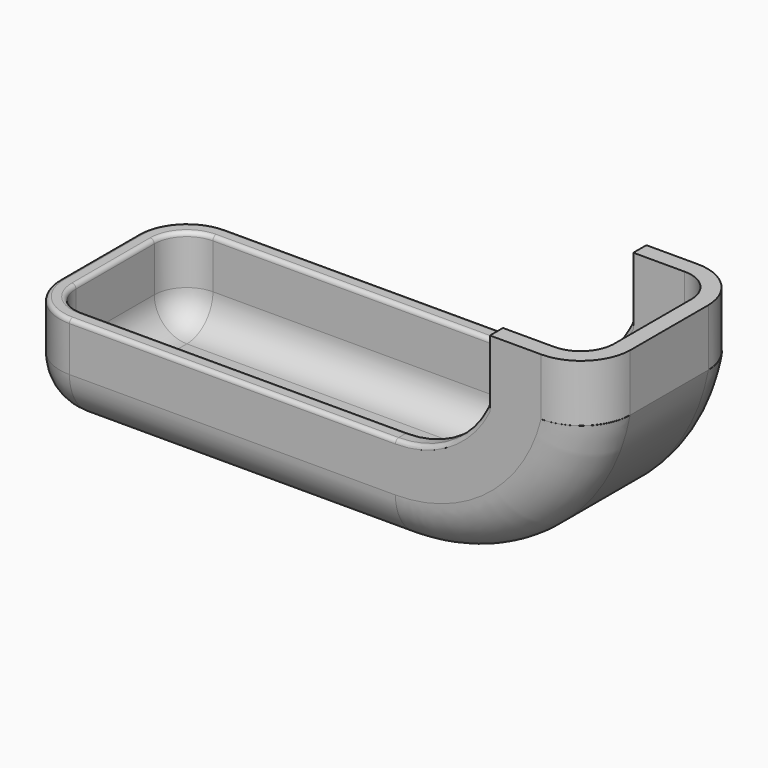
from build123d import *

# Parameters (mm, degrees)
F3_R      = 6
F4_T      = -2
F6_W      = 43.5708351433
F6_H      = 71.2567269802
F7_DEPTH  = 25.2
F9_DEPTH  = 7
F10_W     = 21.0461514253
F10_H     = 5.3538460713
F11_DEPTH = 73.3
F12_R     = 0.5


with BuildPart() as f2:
    # F2: sweep along a path in F0
    with BuildLine(Plane.XZ) as f2_path:
        Line((0, -24.4), (46, -24.4))
        ThreePointArc((46, -24.4), (61.6204993518, -18.7445992222), (70, -4.4))
    # F1 (on Right) → F2 (sweep)
    with BuildSketch(Plane.YZ):
        with BuildLine():
            Line((-6, -24.4), (6, -24.4))
            ThreePointArc((6, -24.4), (10.2426406871, -22.6426406871), (12, -18.4))
            Line((12, -18.4), (12, -12.4))
            Line((12, -12.4), (-12, -12.4))
            Line((-12, -12.4), (-12, -18.4))
            ThreePointArc((-12, -18.4), (-10.2426406871, -22.6426406871), (-6, -24.4))
        make_face()
    sweep(path=f2_path.line)

    # F3
    f3_edges = [f2.edges().sort_by_distance(p)[0] for p in [
        (0, -12, -15.4),
        (0, 10.242641, -22.642641),
        (0, 12, -15.4),
        (0, -10.242641, -22.642641),
    ]]
    fillet(f3_edges, radius=F3_R)

    # F4
    f4_openings = [f2.faces().sort_by_distance(p)[0] for p in [
        (23.307448, 0, -12.4),
        (53.938287, 0, -9.525944),
        (63.838518, 0, -3.270395),
    ]]
    offset(amount=F4_T, openings=f4_openings)

    # F6 (on face) → F7 (cut)
    with BuildSketch(Plane.XY.offset(-4.4)):
        with Locations((56.7423906177, -0.4439689219)):
            Rectangle(F6_W, F6_H)
    extrude(amount=F7_DEPTH, mode=Mode.SUBTRACT)

    # F8 (on face) → F9 (join)
    with BuildSketch(Plane.XY.offset(-4.4)):
        with BuildLine():
            Line((63.8661691473, 12), (57.593101397, 12))
            Line((57.593101397, 12), (57.593101397, 10))
            Line((57.593101397, 10), (63.8661691473, 10))
            ThreePointArc((63.8661691473, 10), (66.7292527517, 8.8342023924), (67.9636062613, 6))
            Line((67.9636062613, 6), (67.9636062613, -6))
            ThreePointArc((67.9636062613, -6), (66.7292527517, -8.8342023924), (63.8661691473, -10))
            Line((63.8661691473, -10), (57.593101397, -10))
            Line((57.593101397, -10), (57.593101397, -12))
            Line((57.593101397, -12), (63.8661691473, -12))
            ThreePointArc((63.8661691473, -12), (68.1563871176, -10.250588481), (70, -6))
            Line((70, -6), (70, 6))
            ThreePointArc((70, 6), (68.1563871176, 10.250588481), (63.8661691473, 12))
        make_face()
    extrude(amount=F9_DEPTH)

    # F10 (on face) → F11 (cut)
    with BuildSketch(Plane(origin=(0, 0, 0), x_dir=(0, -1, 0), z_dir=(-1, 0, 0))):
        with Locations((0.9807674214, -26.6769230357)):
            Rectangle(F10_W, F10_H)
    extrude(amount=-F11_DEPTH, mode=Mode.SUBTRACT)

    # F12
    f12_edges = [f2.edges().sort_by_distance(p)[0] for p in [
        (26, -12, -12.4),
        (53.042727, -12, -10.205881),
        (26, 12, -12.4),
        (1.757359, 10.242641, -12.4),
        (0, 0, -12.4),
        (1.757359, -10.242641, -12.4),
        (26, -10, -12.4),
        (3.171573, -8.828427, -12.4),
        (2, 0, -12.4),
        (3.171573, 8.828427, -12.4),
        (26, 10, -12.4),
        (53.042727, -10, -10.205881),
        (53.042727, 10, -10.205881),
        (53.042727, 12, -10.205881),
    ]]
    fillet(f12_edges, radius=F12_R)


solid = f2.part
